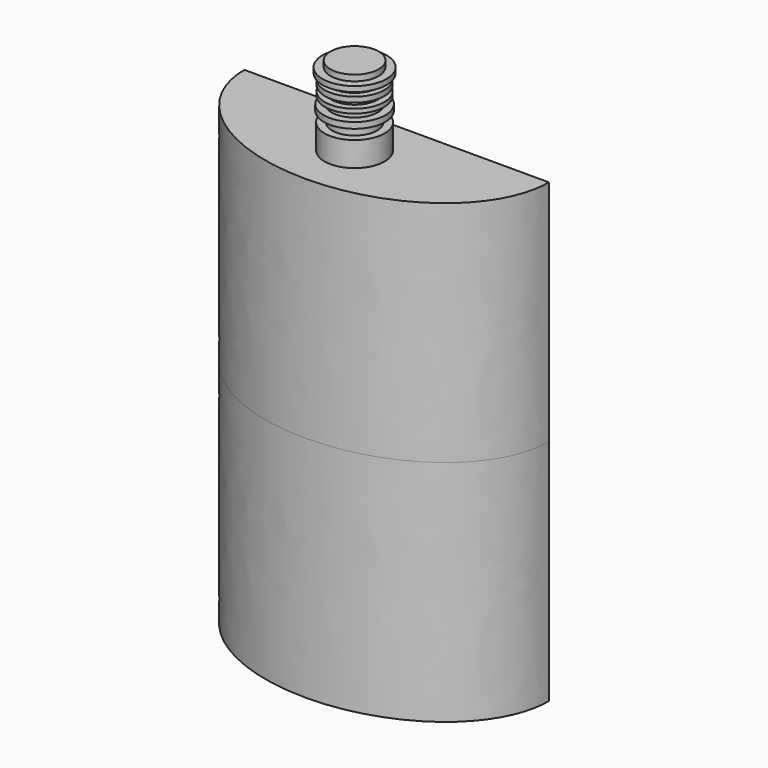
from build123d import *

# Parameters (mm, degrees)
F1_DEPTH      = 76.2
F1_DEPTH_BACK = 76.2


# Not quite as in the source:
# - a feature of the source that left no trace in its solid (it failed there, or was rolled back) is left out


with BuildPart() as f1:
    # F0 (on Top) → F1 (new body, two sides)
    with BuildSketch(Plane.XY) as f1_sk:
        with BuildLine():
            Line((50.8, 0), (-50.8, 0))
            add(Edge.make_bspline(
                [(-50.8, 0), (-50.8, -38.1), (0, -38.1), (50.8, -38.1), (50.8, 0)],
                knots=[0, 0, 0, 1.5707963268, 1.5707963268, 3.1415926536, 3.1415926536, 3.1415926536], degree=2, weights=[1, 0.7071067812, 1, 0.7071067812, 1]))
        make_face()
    extrude(amount=F1_DEPTH)
    extrude(f1_sk.sketch, amount=-F1_DEPTH_BACK)

    # F2 (on Right) → F3 (revolve)
    with BuildSketch(Plane.YZ):
        Polygon((-27.5835152715, 76.0684758425), (-17.5483282655, 76.2890353799), (-17.5483282655, 102.6451811194), (-25.5985315889, 102.6451811194), (-25.5985315889, 100.6601974368), (-28.2451752573, 100.6601974368), (-28.2451752573, 98.8957732916), (-25.3779776394, 98.8957732916), (-25.3779776394, 97.1313416958), (-27.4732373655, 97.1313416958), (-27.4732373655, 95.3669101), (-25.267701596, 95.3669101), (-25.267701596, 93.6024859548), (-27.4732373655, 93.6024859548), (-27.4732373655, 92.1688899398), (-25.267701596, 92.1688899398), (-25.267701596, 89.8530781269), (-27.8040673584, 89.8530781269), (-27.8040673584, 87.8680944443), (-25.0471476465, 87.8680944443), (-25.0471476465, 84.4495147467), (-27.5835152715, 84.4495147467), align=None)
    revolve(axis=Axis((0, -17.5483282655, 90.2941823006), (0, 0, -1)))


solid = f1.part
